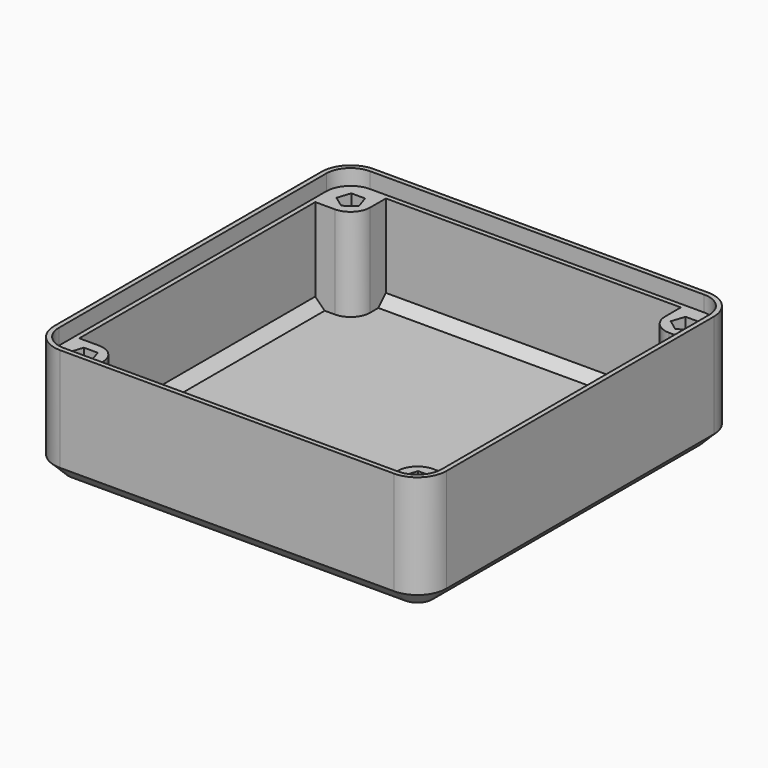
from build123d import *

# Parameters (mm, degrees)
F3_DEPTH  = 13
F4_T      = -1.2
F6_SIZE   = 1.8
F7_SIZE   = 1.2
F8_DEPTH  = 11.8
F10_DEPTH = 2


# Not quite as in the source:
# - a feature names something its author has since deleted; it is built from what else it names


with BuildPart() as f3:
    # F2 (on Top) → F3 (new body)
    with BuildSketch(Plane.XY):
        with BuildLine():
            ThreePointArc((-25, -21.3), (-23.9162950904, -23.9162950904), (-21.3, -25))
            Line((-21.3, -25), (21.3, -25))
            ThreePointArc((21.3, -25), (23.9162950904, -23.9162950904), (25, -21.3))
            Line((25, -21.3), (25, 21.3))
            ThreePointArc((25, 21.3), (23.9162950904, 23.9162950904), (21.3, 25))
            Line((21.3, 25), (-21.3, 25))
            ThreePointArc((-21.3, 25), (-23.9162950904, 23.9162950904), (-25, 21.3))
            Line((-25, 21.3), (-25, -21.3))
        make_face()
    extrude(amount=F3_DEPTH)

    # F4
    f4_openings = [f3.faces().sort_by_distance(p)[0] for p in [
        (0, 0, 13),
    ]]
    offset(amount=F4_T, openings=f4_openings)

    # F6
    f6_edges = [f3.edges().sort_by_distance(p)[0] for p in [
        (-23.916295, -23.916295, 0),
        (0, -25, 0),
        (23.916295, -23.916295, 0),
        (25, 0, 0),
        (23.916295, 23.916295, 0),
        (0, 25, 0),
        (-23.916295, 23.916295, 0),
        (-25, 0, 0),
    ]]
    chamfer(f6_edges, length=F6_SIZE)

    # F7
    f7_edges = [f3.edges().sort_by_distance(p)[0] for p in [
        (-23.067767, -23.067767, 1.2),
        (0, -23.8, 1.2),
        (23.067767, -23.067767, 1.2),
        (23.8, 0, 1.2),
        (23.067767, 23.067767, 1.2),
        (0, 23.8, 1.2),
        (-23.067767, 23.067767, 1.2),
        (-23.8, 0, 1.2),
    ]]
    chamfer(f7_edges, length=F7_SIZE)

    # F5 (on face) → F8 (join, through all)
    with BuildSketch(Plane.XY.offset(1.2)):
        with BuildLine():
            Line((-23.8, 18.8), (-21.3, 18.8))
            ThreePointArc((-21.3, 18.8), (-19.532233047, 19.532233047), (-18.8, 21.3))
            Line((-18.8, 21.3), (-18.8, 23.8))
            Line((-18.8, 23.8), (-21.3, 23.8))
            ThreePointArc((-21.3, 23.8), (-23.067766953, 23.067766953), (-23.8, 21.3))
            Line((-23.8, 21.3), (-23.8, 18.8))
        make_face()
        Polygon((-19.8734152256, 20.8364745084), (-21.3, 19.8), (-22.7265847744, 20.8364745084), (-22.1816778784, 22.5135254916), (-20.4183221216, 22.5135254916), align=None, mode=Mode.SUBTRACT)
        with BuildLine():
            Line((-21.3, -18.8), (-23.8, -18.8))
            Line((-23.8, -18.8), (-23.8, -21.3))
            ThreePointArc((-23.8, -21.3), (-23.067766953, -23.067766953), (-21.3, -23.8))
            Line((-21.3, -23.8), (-18.8, -23.8))
            Line((-18.8, -23.8), (-18.8, -21.3))
            ThreePointArc((-18.8, -21.3), (-19.532233047, -19.532233047), (-21.3, -18.8))
        make_face()
        Polygon((-22.7265847744, -21.7635254916), (-22.1816778784, -20.0864745084), (-20.4183221216, -20.0864745084), (-19.8734152256, -21.7635254916), (-21.3, -22.8), align=None, mode=Mode.SUBTRACT)
        with BuildLine():
            Line((21.3, 23.8), (18.8, 23.8))
            Line((18.8, 23.8), (18.8, 21.3))
            ThreePointArc((18.8, 21.3), (19.532233047, 19.532233047), (21.3, 18.8))
            Line((21.3, 18.8), (23.8, 18.8))
            Line((23.8, 18.8), (23.8, 21.3))
            ThreePointArc((23.8, 21.3), (23.067766953, 23.067766953), (21.3, 23.8))
        make_face()
        Polygon((19.8734152256, 20.8364745084), (20.4183221216, 22.5135254916), (22.1816778784, 22.5135254916), (22.7265847744, 20.8364745084), (21.3, 19.8), align=None, mode=Mode.SUBTRACT)
        with BuildLine():
            Line((18.8, -21.3), (18.8, -23.8))
            Line((18.8, -23.8), (21.3, -23.8))
            ThreePointArc((21.3, -23.8), (23.067766953, -23.067766953), (23.8, -21.3))
            Line((23.8, -21.3), (23.8, -18.8))
            Line((23.8, -18.8), (21.3, -18.8))
            ThreePointArc((21.3, -18.8), (19.532233047, -19.532233047), (18.8, -21.3))
        make_face()
        Polygon((19.8734152256, -21.7635254916), (20.4183221216, -20.0864745084), (22.1816778784, -20.0864745084), (22.7265847744, -21.7635254916), (21.3, -22.8), align=None, mode=Mode.SUBTRACT)
    extrude(amount=F8_DEPTH)

    # F9 (on face) → F10 (join)
    with BuildSketch(Plane.XY.offset(13)):
        with BuildLine():
            Line((-25, 21.3), (-25, -21.3))
            ThreePointArc((-25, -21.3), (-23.9162950904, -23.9162950904), (-21.3, -25))
            Line((-21.3, -25), (21.3, -25))
            ThreePointArc((21.3, -25), (23.9162950904, -23.9162950904), (25, -21.3))
            Line((25, -21.3), (25, 21.3))
            ThreePointArc((25, 21.3), (23.9162950904, 23.9162950904), (21.3, 25))
            Line((21.3, 25), (-21.3, 25))
            ThreePointArc((-21.3, 25), (-23.9162950904, 23.9162950904), (-25, 21.3))
        make_face()
        with BuildLine():
            ThreePointArc((-24.4, 21.3), (-23.4920310217, 23.4920310217), (-21.3, 24.4))
            Line((-21.3, 24.4), (21.3, 24.4))
            ThreePointArc((21.3, 24.4), (23.4920310217, 23.4920310217), (24.4, 21.3))
            Line((24.4, 21.3), (24.4, -21.3))
            ThreePointArc((24.4, -21.3), (23.4920310217, -23.4920310217), (21.3, -24.4))
            Line((21.3, -24.4), (-21.3, -24.4))
            ThreePointArc((-21.3, -24.4), (-23.4920310217, -23.4920310217), (-24.4, -21.3))
            Line((-24.4, -21.3), (-24.4, 21.3))
        make_face(mode=Mode.SUBTRACT)
    extrude(amount=F10_DEPTH)


solid = f3.part
